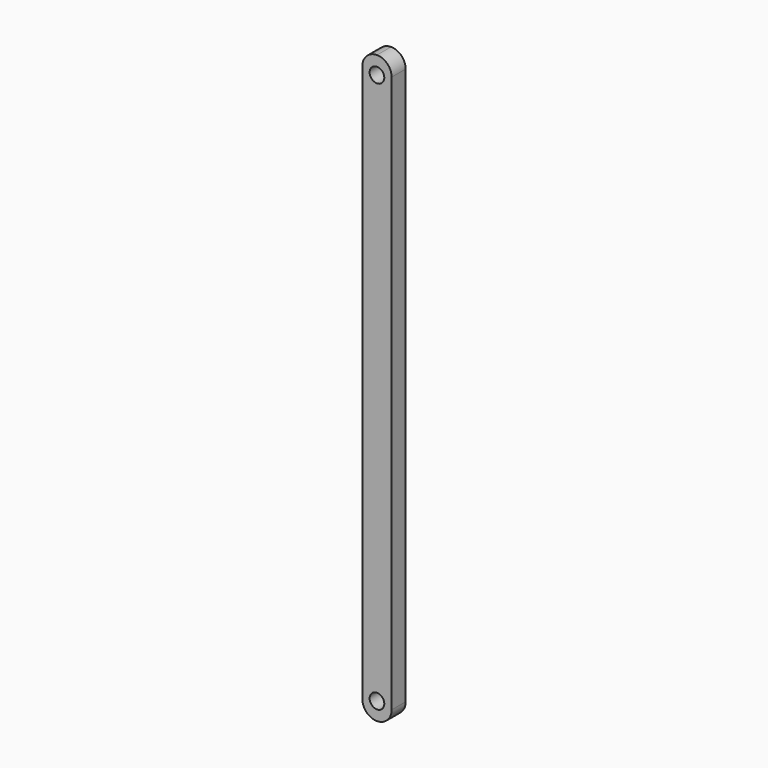
from build123d import *

# Parameters (mm, degrees)
F0_W     = 10
F0_H     = 200
F0_R     = 2.5
F1_DEPTH = 6
F2_R     = 4.99999


# Not quite as in the source:
# - a fillet or chamfer is up to 0.001 mm smaller than in the source, because OpenCascade refuses the exact size


with BuildPart() as f1:
    # F0 (on Front) → F1 (new body)
    with BuildSketch(Plane.XZ):
        Rectangle(F0_W, F0_H)
        with Locations((0, -94)):
            Circle(F0_R, mode=Mode.SUBTRACT)
        with Locations((0, 94)):
            Circle(F0_R, mode=Mode.SUBTRACT)
    extrude(amount=F1_DEPTH)

    # F2 (radius 5 in the source; OpenCascade refuses exactly that, so slightly less here)
    f2_edges = [f1.edges().sort_by_distance(p)[0] for p in [
        (-5, -3, 100),
        (5, -3, 100),
        (5, -3, -100),
        (-5, -3, -100),
    ]]
    fillet(f2_edges, radius=F2_R)


solid = f1.part
